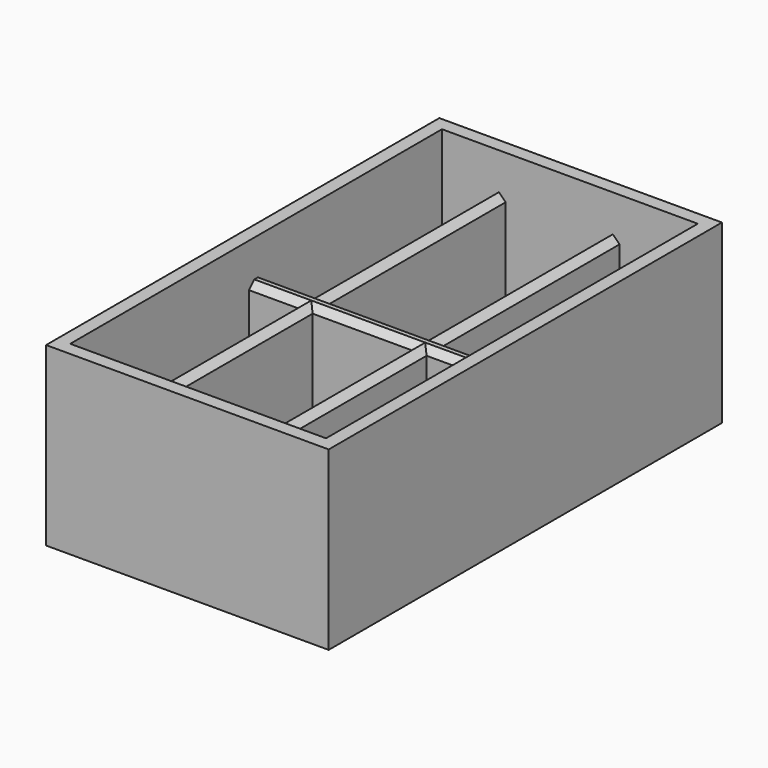
from build123d import *

# Parameters (mm, degrees)
F0_W     = 2.4
F0_H     = 40
F0_H_2   = 3.2
F1_DEPTH = 31.6
F0_W_2   = 9
F0_W_3   = 18
F0_W_4   = 14
F2_DEPTH = 2.4
F3_DEPTH = 25
F4_SIZE  = 1.19999


# Not quite as in the source:
# - a fillet or chamfer is up to 0.001 mm smaller than in the source, because OpenCascade refuses the exact size


with BuildPart() as f1:
    # F0 (on Top) → F1 (new body)
    with BuildSketch(Plane.XY):
        Polygon((-9.4000064151, 44), (-60.0000064151, 44), (-60.0000064151, -44), (-9.4000064151, -44), (-9.4000064151, -41.6), (-11.8000064151, -41.6), (-25.8000064151, -41.6), (-28.2000064151, -41.6), (-46.2000064151, -41.6), (-48.6000064151, -41.6), (-57.6000064151, -41.6), (-57.6000064151, -1.6), (-57.6000064151, 1.6), (-57.6000064151, 41.6), (-48.6000064151, 41.6), (-46.2000064151, 41.6), (-28.2000064151, 41.6), (-25.8000064151, 41.6), (-11.8000064151, 41.6), (-9.4000064151, 41.6), align=None)
        with Locations((-10.6000064151, 21.6)):
            Rectangle(F0_W, F0_H)
        with Locations((-10.6000064151, 0)):
            Rectangle(F0_W, F0_H_2)
        with Locations((-10.6000064151, -21.6)):
            Rectangle(F0_W, F0_H)
    extrude(amount=F1_DEPTH)

    # F0 (on Top) → F2 (join)
    with BuildSketch(Plane.XY):
        with Locations((-53.1000064151, 21.6)):
            Rectangle(F0_W_2, F0_H)
        with Locations((-53.1000064151, 0)):
            Rectangle(F0_W_2, F0_H_2)
        with Locations((-53.1000064151, -21.6)):
            Rectangle(F0_W_2, F0_H)
        with Locations((-37.2000064151, 21.6)):
            Rectangle(F0_W_3, F0_H)
        with Locations((-37.2000064151, 0)):
            Rectangle(F0_W_3, F0_H_2)
        with Locations((-37.2000064151, -21.6)):
            Rectangle(F0_W_3, F0_H)
        with Locations((-18.8000064151, 21.6)):
            Rectangle(F0_W_4, F0_H)
        with Locations((-18.8000064151, 0)):
            Rectangle(F0_W_4, F0_H_2)
        with Locations((-18.8000064151, -21.6)):
            Rectangle(F0_W_4, F0_H)
    extrude(amount=F2_DEPTH)

    # F0 (on Top) → F3 (join)
    with BuildSketch(Plane.XY):
        Polygon((-9.4000064151, 44), (-60.0000064151, 44), (-60.0000064151, -44), (-9.4000064151, -44), (-9.4000064151, -41.6), (-11.8000064151, -41.6), (-25.8000064151, -41.6), (-28.2000064151, -41.6), (-46.2000064151, -41.6), (-48.6000064151, -41.6), (-57.6000064151, -41.6), (-57.6000064151, -1.6), (-57.6000064151, 1.6), (-57.6000064151, 41.6), (-48.6000064151, 41.6), (-46.2000064151, 41.6), (-28.2000064151, 41.6), (-25.8000064151, 41.6), (-11.8000064151, 41.6), (-9.4000064151, 41.6), align=None)
        with Locations((-10.6000064151, 21.6)):
            Rectangle(F0_W, F0_H)
        with Locations((-10.6000064151, -21.6)):
            Rectangle(F0_W, F0_H)
        with Locations((-10.6000064151, 0)):
            Rectangle(F0_W, F0_H_2)
        with Locations((-53.1000064151, 0)):
            Rectangle(F0_W_2, F0_H_2)
        with Locations((-47.4000064151, 0)):
            Rectangle(F0_W, F0_H_2)
        with Locations((-47.4000064151, 21.6)):
            Rectangle(F0_W, F0_H)
        with Locations((-47.4000064151, -21.6)):
            Rectangle(F0_W, F0_H)
        with Locations((-37.2000064151, 0)):
            Rectangle(F0_W_3, F0_H_2)
        with Locations((-27.0000064151, 21.6)):
            Rectangle(F0_W, F0_H)
        with Locations((-27.0000064151, 0)):
            Rectangle(F0_W, F0_H_2)
        with Locations((-18.8000064151, 0)):
            Rectangle(F0_W_4, F0_H_2)
        with Locations((-27.0000064151, -21.6)):
            Rectangle(F0_W, F0_H)
    extrude(amount=F3_DEPTH)

    # F4 (size 1.2 in the source; OpenCascade refuses exactly that, so slightly less here)
    f4_edges = [f1.edges().sort_by_distance(p)[0] for p in [
        (-53.100006, 1.6, 25),
        (-53.100006, -1.6, 25),
        (-46.200006, -21.6, 25),
        (-48.600006, -21.6, 25),
        (-48.600006, 21.6, 25),
        (-46.200006, 21.6, 25),
        (-37.200006, 1.6, 25),
        (-37.200006, -1.6, 25),
        (-28.200006, -21.6, 25),
        (-25.800006, -21.6, 25),
        (-18.800006, -1.6, 25),
        (-18.800006, 1.6, 25),
        (-25.800006, 21.6, 25),
        (-28.200006, 21.6, 25),
    ]]
    chamfer(f4_edges, length=F4_SIZE)


solid = f1.part
